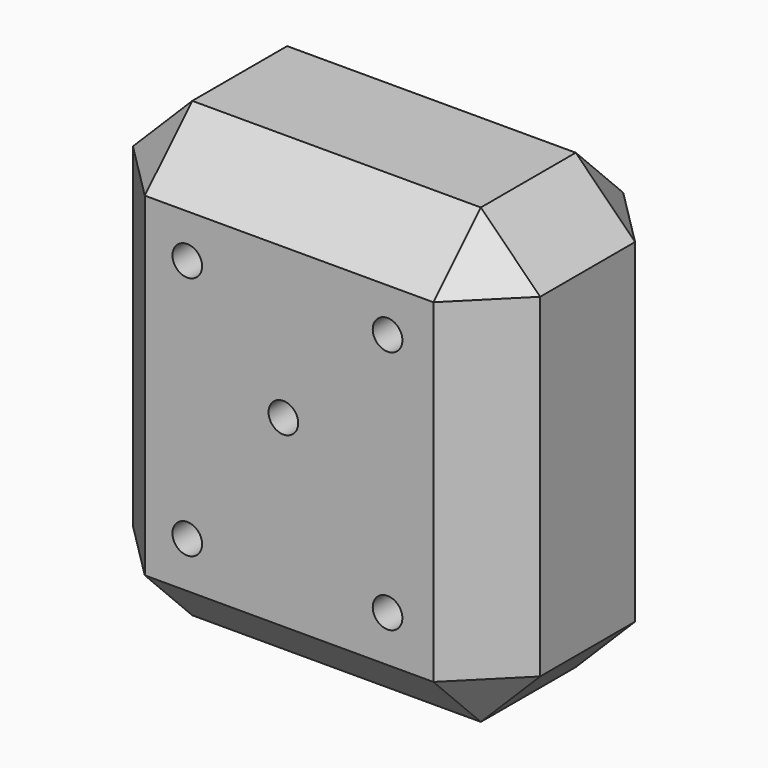
from build123d import *

# Parameters (mm, degrees)
F0_W           = 87.1929600835
F0_H           = 96.9703122973
F1_DEPTH       = 50.8
F3_D           = 6.35
F3_CBORE_D     = 12.7
F3_CBORE_DEPTH = 25.4
F5_D           = 6.35
F5_CSINK_D     = 12.7
F5_CSINK_ANGLE = 90
F6_SIZE        = 12.7


# Not quite as in the source:
# - a feature names something its author has since deleted; it is built from what else it names


with BuildPart() as f1:
    # F0 (on Front) → F1 (new body)
    with BuildSketch(Plane.XZ):
        with Locations((1.2225024402, -3.5745240748)):
            Rectangle(F0_W, F0_H)
    extrude(amount=F1_DEPTH)

    # F3 (through all)
    with Locations(Plane(origin=(0, 0, 0), x_dir=(1, 0, 0), z_dir=(0, 1, 0))):
        with Locations((0, 0)):
            CounterBoreHole(F3_D / 2, F3_CBORE_D / 2, F3_CBORE_DEPTH)

    # F5 (through all)
    with Locations(Plane(origin=(0, 0, 0), x_dir=(1, 0, 0), z_dir=(0, 1, 0))):
        with Locations((22.3049465567, -22.8805579245), (-20.5781124532, -22.8805579245), (-20.5781124532, 29.5000895858), (22.3049465567, 29.5000895858)):
            CounterSinkHole(F5_D / 2, F5_CSINK_D / 2, counter_sink_angle=F5_CSINK_ANGLE)

    # F6
    f6_edges = [f1.edges().sort_by_distance(p)[0] for p in [
        (-42.373978, -25.4, -52.05968),
        (44.818982, -25.4, -52.05968),
        (1.222502, 0, -52.05968),
        (1.222502, -50.8, -52.05968),
        (-42.373978, -25.4, 44.910632),
        (-42.373978, 0, -3.574524),
        (-42.373978, -50.8, -3.574524),
        (44.818982, -25.4, 44.910632),
        (44.818982, 0, -3.574524),
        (44.818982, -50.8, -3.574524),
        (1.222502, 0, 44.910632),
        (1.222502, -50.8, 44.910632),
    ]]
    chamfer(f6_edges, length=F6_SIZE)


solid = f1.part
